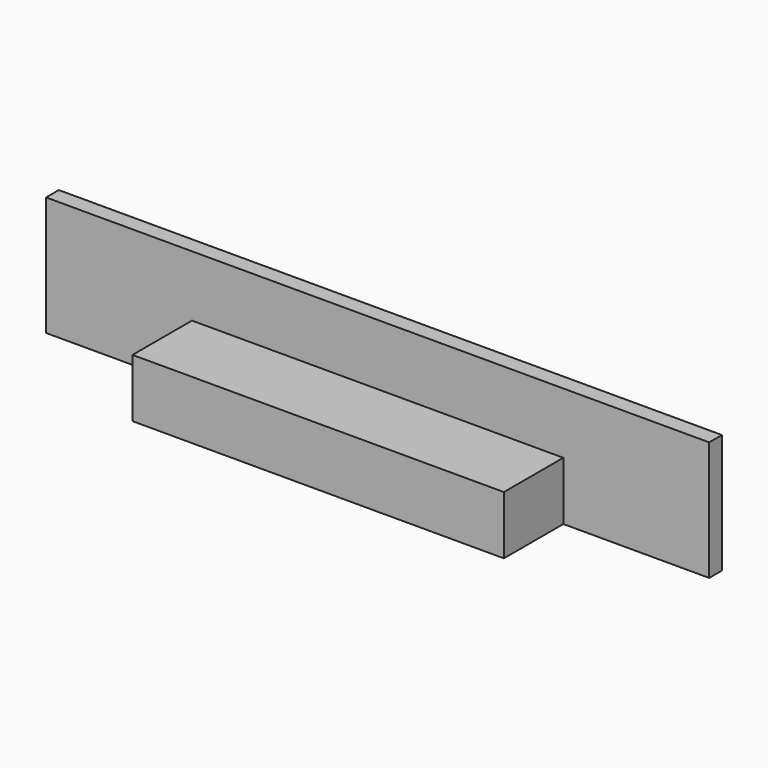
from build123d import *

# Parameters (mm, degrees)
F0_W         = 250
F0_H         = 45
F1_DEPTH     = 6
F2_W         = 140
F2_H         = 22
F3_DEPTH     = 28
F4_TEXT_SIZE = 19.4444444444
F5_DEPTH     = 0.2


# Not quite as in the source:
# - Text() gives the source's letters only with a copy of the font that has no kerning and outlines rounded to 1/6400 em; it was checked with that copy


with BuildPart() as f1:
    # F0 (on Front) → F1 (new body)
    with BuildSketch(Plane.XZ):
        Rectangle(F0_W, F0_H)
    extrude(amount=F1_DEPTH)

    # F2 (on face) → F3 (join)
    with BuildSketch(Plane.XZ.offset(6)):
        with Locations((0, -11.5)):
            Rectangle(F2_W, F2_H)
    extrude(amount=F3_DEPTH)

    # F4 (on face) → F5 (join)
    with BuildSketch(Plane(origin=(0, 0, 0), x_dir=(-1, 0, 0), z_dir=(0, 1, 0))):
        with Locations((-117.0889756944, -5.7684085158)):
            Text('REMOVE BEFORE FLIGHT', F4_TEXT_SIZE, font='Open Sans', font_style=FontStyle.BOLD, text_align=(TextAlign.LEFT, TextAlign.BOTTOM))
    extrude(amount=F5_DEPTH)


solid = f1.part
